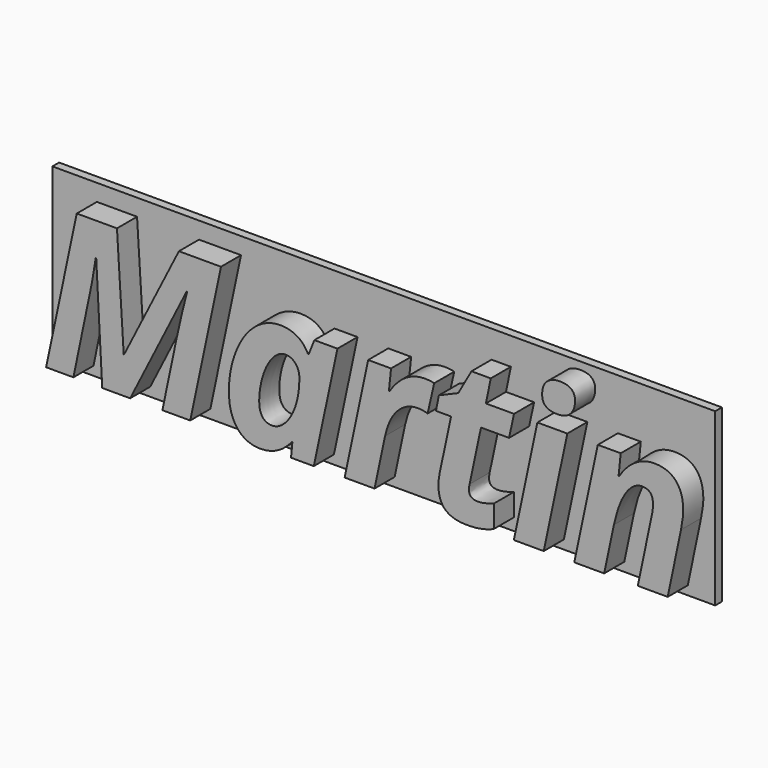
from build123d import *

# Parameters (mm, degrees)
F0_TEXT_SIZE = 24.314187174
F1_DEPTH     = 3
F2_W         = 79.1520364583
F2_H         = 20.4215215053
F3_DEPTH     = 1


# Not quite as in the source:
# - Text() gives the source's letters only with a copy of the font that has no kerning and outlines rounded to 1/6400 em; it was checked with that copy


with BuildPart() as f1:
    # F0 (on Front) → F1 (new body)
    with BuildSketch(Plane.XZ):
        with Locations((-44.7518088037, -0.1232831214)):
            Text('Martin', F0_TEXT_SIZE, font='Open Sans', font_style=FontStyle.BOLDITALIC, text_align=(TextAlign.LEFT, TextAlign.BOTTOM))
    extrude(amount=F1_DEPTH)

    # F2 (on face) → F3 (join)
    with BuildSketch(Plane.XZ):
        with Locations((-6.1896089464, 9.0292982059)):
            Rectangle(F2_W, F2_H)
    extrude(amount=-F3_DEPTH)


solid = f1.part
